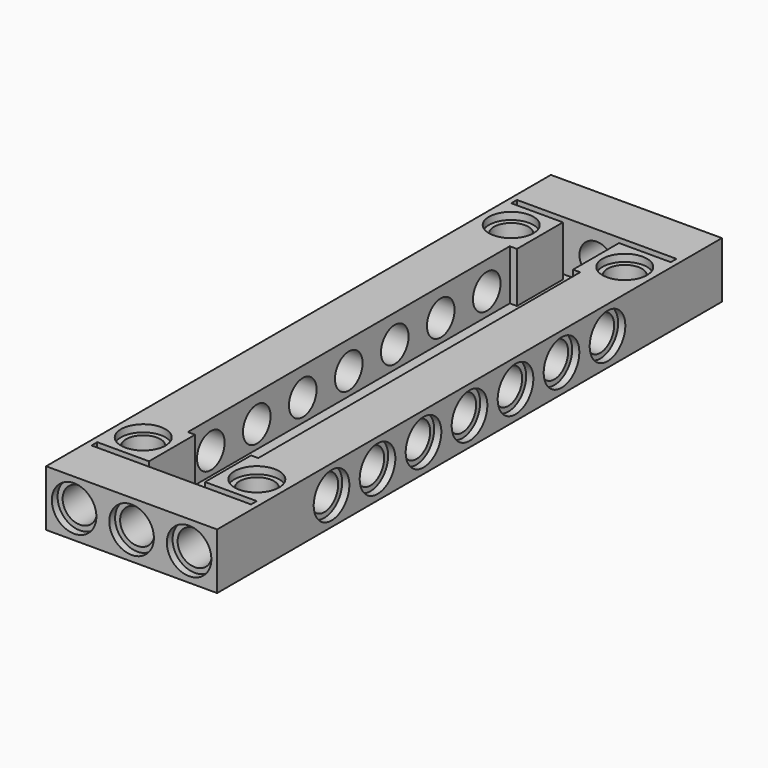
from build123d import *

# Parameters (mm, degrees)
F0_R      = 3.1
F0_R_2    = 2.4
F1_DEPTH  = 87.8
F2_DEPTH  = 1
F3_DEPTH  = 8
F4_R      = 2.4
F5_DEPTH  = 25
F4_R_2    = 3.1
F6_DEPTH  = 1
F7_R      = 3.1
F7_R_2    = 2.4
F8_DEPTH  = 1
F9_R      = 2.4
F10_DEPTH = 8
F9_R_2    = 3.1
F11_DEPTH = 1
F12_DEPTH = 7
F13_R     = 2.4
F14_DEPTH = 7.9
F13_R_2   = 3.1
F15_DEPTH = 1


# Not quite as in the source:
# - a pattern or mirror of a feature is missing from the dataset's text; its kind, count and spacing are read off the source's solid


with BuildPart() as f1:
    # F0 (on Front) → F1 (new body)
    with BuildSketch(Plane.XZ):
        Polygon((4, 7.8), (0, 7.8), (-4, 7.8), (-11.9, 7.8), (-11.9, 0), (0, 0), (11.9, 0), (11.9, 7.8), align=None)
        with Locations((-7.975, 3.9)):
            Circle(F0_R, mode=Mode.SUBTRACT)
        with Locations((0, 3.9)):
            Circle(F0_R, mode=Mode.SUBTRACT)
        with Locations((7.975, 3.9)):
            Circle(F0_R, mode=Mode.SUBTRACT)
        with Locations((7.975, 3.9)):
            Circle(F0_R)
        with Locations((7.975, 3.9)):
            Circle(F0_R_2, mode=Mode.SUBTRACT)
        with Locations((0, 3.9)):
            Circle(F0_R)
        with Locations((0, 3.9)):
            Circle(F0_R_2, mode=Mode.SUBTRACT)
        with Locations((-7.975, 3.9)):
            Circle(F0_R)
        with Locations((-7.975, 3.9)):
            Circle(F0_R_2, mode=Mode.SUBTRACT)
        with Locations((-7.975, 3.9)):
            Circle(F0_R_2)
        with Locations((0, 3.9)):
            Circle(F0_R_2)
        with Locations((7.975, 3.9)):
            Circle(F0_R_2)
    extrude(amount=F1_DEPTH)

    # F0 (on Front) → F2 (cut)
    with BuildSketch(Plane.XZ):
        with Locations((7.975, 3.9)):
            Circle(F0_R)
        with Locations((7.975, 3.9)):
            Circle(F0_R_2, mode=Mode.SUBTRACT)
        with Locations((0, 3.9)):
            Circle(F0_R)
        with Locations((0, 3.9)):
            Circle(F0_R_2, mode=Mode.SUBTRACT)
        with Locations((-7.975, 3.9)):
            Circle(F0_R)
        with Locations((-7.975, 3.9)):
            Circle(F0_R_2, mode=Mode.SUBTRACT)
    extrude(amount=F2_DEPTH, mode=Mode.SUBTRACT)

    # F0 (on Front) → F3 (cut)
    with BuildSketch(Plane.XZ):
        with Locations((-7.975, 3.9)):
            Circle(F0_R_2)
        with Locations((0, 3.9)):
            Circle(F0_R_2)
        with Locations((7.975, 3.9)):
            Circle(F0_R_2)
    extrude(amount=F3_DEPTH, mode=Mode.SUBTRACT)

    # F4 (on face) → F5 (cut)
    with BuildSketch(Plane.XY.offset(7.8)):
        with Locations((-7.9, -11.9)):
            Circle(F4_R)
        with Locations((-7.9, -75.9)):
            Circle(F4_R)
        with Locations((7.9, -75.9)):
            Circle(F4_R)
        with Locations((7.9, -11.9)):
            Circle(F4_R)
    extrude(amount=-F5_DEPTH, mode=Mode.SUBTRACT)

    # F4 (on face) → F6 (cut)
    with BuildSketch(Plane.XY.offset(7.8)):
        with Locations((-7.9, -11.9)):
            Circle(F4_R_2)
        with Locations((-7.9, -11.9)):
            Circle(F4_R, mode=Mode.SUBTRACT)
        with Locations((7.9, -11.9)):
            Circle(F4_R_2)
        with Locations((7.9, -11.9)):
            Circle(F4_R, mode=Mode.SUBTRACT)
        with Locations((-7.9, -75.9)):
            Circle(F4_R_2)
        with Locations((-7.9, -75.9)):
            Circle(F4_R, mode=Mode.SUBTRACT)
        with Locations((7.9, -75.9)):
            Circle(F4_R_2)
        with Locations((7.9, -75.9)):
            Circle(F4_R, mode=Mode.SUBTRACT)
    extrude(amount=-F6_DEPTH, mode=Mode.SUBTRACT)

    # F7 (on face) → F8 (cut)
    with BuildSketch(Plane(origin=(0, 0, 0), x_dir=(1, 0, 0), z_dir=(0, 0, -1))):
        with Locations((7.9, 75.9)):
            Circle(F7_R)
        with Locations((7.9, 75.9)):
            Circle(F7_R_2, mode=Mode.SUBTRACT)
        with Locations((-7.9, 75.9)):
            Circle(F7_R)
        with Locations((-7.9, 75.9)):
            Circle(F7_R_2, mode=Mode.SUBTRACT)
        with Locations((-7.9, 11.9)):
            Circle(F7_R)
        with Locations((-7.9, 11.9)):
            Circle(F7_R_2, mode=Mode.SUBTRACT)
        with Locations((7.9, 11.9)):
            Circle(F7_R)
        with Locations((7.9, 11.9)):
            Circle(F7_R_2, mode=Mode.SUBTRACT)
    extrude(amount=-F8_DEPTH, mode=Mode.SUBTRACT)

    # F9 (on face) → F10 (cut)
    with BuildSketch(Plane.YZ.offset(11.9)):
        with Locations((-67.9, 3.9)):
            Circle(F9_R)
        with Locations((-59.9, 3.9)):
            Circle(F9_R)
        with Locations((-51.9, 3.9)):
            Circle(F9_R)
        with Locations((-43.9, 3.9)):
            Circle(F9_R)
        with Locations((-35.9, 3.9)):
            Circle(F9_R)
        with Locations((-27.9, 3.9)):
            Circle(F9_R)
        with Locations((-19.9, 3.9)):
            Circle(F9_R)
    f10 = extrude(amount=-F10_DEPTH, mode=Mode.SUBTRACT)

    # F10_copies: F10 across plane
    add(f10.mirror(Plane(origin=(0, 0, 0), x_dir=(0, 0, -1), z_dir=(-1, 0, 0))), mode=Mode.SUBTRACT)

    # F9 (on face) → F11 (cut)
    with BuildSketch(Plane.YZ.offset(11.9)):
        with Locations((-67.9, 3.9)):
            Circle(F9_R_2)
        with Locations((-67.9, 3.9)):
            Circle(F9_R, mode=Mode.SUBTRACT)
        with Locations((-59.9, 3.9)):
            Circle(F9_R_2)
        with Locations((-59.9, 3.9)):
            Circle(F9_R, mode=Mode.SUBTRACT)
        with Locations((-51.9, 3.9)):
            Circle(F9_R_2)
        with Locations((-51.9, 3.9)):
            Circle(F9_R, mode=Mode.SUBTRACT)
        with Locations((-43.9, 3.9)):
            Circle(F9_R_2)
        with Locations((-43.9, 3.9)):
            Circle(F9_R, mode=Mode.SUBTRACT)
        with Locations((-35.9, 3.9)):
            Circle(F9_R_2)
        with Locations((-35.9, 3.9)):
            Circle(F9_R, mode=Mode.SUBTRACT)
        with Locations((-27.9, 3.9)):
            Circle(F9_R_2)
        with Locations((-27.9, 3.9)):
            Circle(F9_R, mode=Mode.SUBTRACT)
        with Locations((-19.9, 3.9)):
            Circle(F9_R_2)
        with Locations((-19.9, 3.9)):
            Circle(F9_R, mode=Mode.SUBTRACT)
    f11 = extrude(amount=-F11_DEPTH, mode=Mode.SUBTRACT)

    # F11_copies: F11 across plane
    add(f11.mirror(Plane(origin=(0, 0, 0), x_dir=(0, 0, -1), z_dir=(-1, 0, 0))), mode=Mode.SUBTRACT)

    # F4 (on face) → F12 (cut)
    with BuildSketch(Plane.XY.offset(7.8)):
        Polygon((-11.1, -6.9), (-11.1, -7.9), (-3.9, -7.9), (-3.9, -15.9), (-4.9, -15.9), (-4.9, -71.9), (-3.9, -71.9), (-3.9, -79.9), (-11.1, -79.9), (-11.1, -80.9), (11.1, -80.9), (11.1, -79.9), (3.9, -79.9), (3.9, -71.9), (4.9, -71.9), (4.9, -15.9), (3.9, -15.9), (3.9, -7.9), (11.1, -7.9), (11.1, -6.9), align=None)
    extrude(amount=-F12_DEPTH, mode=Mode.SUBTRACT)

    # F13 (on face) → F14 (cut)
    with BuildSketch(Plane.XZ.offset(87.8)):
        with Locations((-8, 3.9)):
            Circle(F13_R)
        with Locations((0, 3.9)):
            Circle(F13_R)
        with Locations((8, 3.9)):
            Circle(F13_R)
    extrude(amount=-F14_DEPTH, mode=Mode.SUBTRACT)

    # F13 (on face) → F15 (cut)
    with BuildSketch(Plane.XZ.offset(87.8)):
        with Locations((-8, 3.9)):
            Circle(F13_R_2)
        with Locations((-8, 3.9)):
            Circle(F13_R, mode=Mode.SUBTRACT)
        with Locations((0, 3.9)):
            Circle(F13_R_2)
        with Locations((0, 3.9)):
            Circle(F13_R, mode=Mode.SUBTRACT)
        with Locations((8, 3.9)):
            Circle(F13_R_2)
        with Locations((8, 3.9)):
            Circle(F13_R, mode=Mode.SUBTRACT)
    extrude(amount=-F15_DEPTH, mode=Mode.SUBTRACT)


solid = f1.part
